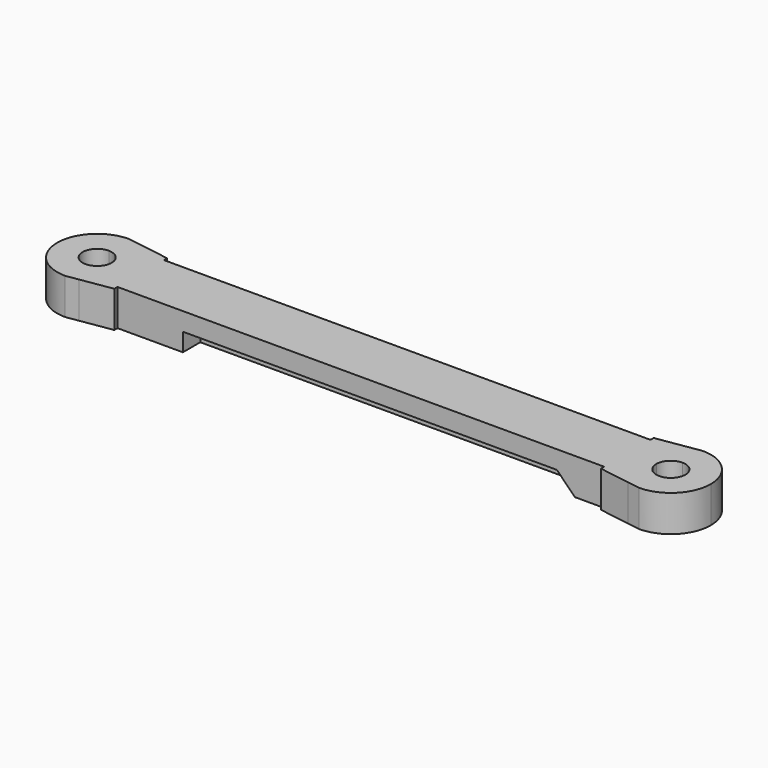
from build123d import *

# Parameters (mm, degrees)
F0_W         = 60
F0_H         = 2
F1_DEPTH     = 5
F2_W         = 9
F2_H         = 3
F3_DEPTH     = 5
F4_W         = 49
F4_H         = 3
F5_DEPTH     = 2.5
F6_T4_DEPTH  = 15.8584149398
F6_T9_DEPTH  = 28.7168298797
F6_T15_DEPTH = 28.7168298797
F6_T21_DEPTH = 15.8584149398


# Not quite as in the source:
# - a fillet or chamfer that OpenCascade refuses, or shapes differently, is made with other operations: its cross-section is extruded or revolved along the edge and cut away or added


with BuildPart() as f1:
    # F0 (on Top) → F1 (new body)
    with BuildSketch(Plane.XY):
        with BuildLine():
            ThreePointArc((21.3155073225, 23.6537444443), (19.7045946191, 27.5428317408), (15.8155073225, 29.1537444443))
            Line((15.8155073225, 29.1537444443), (15.8155073225, 25.6537444443))
            ThreePointArc((15.8155073225, 25.6537444443), (17.2297208849, 25.0679580066), (17.8155073225, 23.6537444443))
            ThreePointArc((17.8155073225, 23.6537444443), (17.2297208849, 22.2395308819), (15.8155073225, 21.6537444443))
            Line((15.8155073225, 21.6537444443), (15.8155073225, 18.1537444443))
            ThreePointArc((15.8155073225, 18.1537444443), (19.7045946191, 19.7646571477), (21.3155073225, 23.6537444443))
        make_face()
        with BuildLine():
            Line((15.8155073225, 29.1537444443), (14.120912728, 28.8861768767))
            ThreePointArc((14.120912728, 28.8861768767), (11.3674588589, 26.8886887815), (10.3155073225, 23.6537444443))
            Line((10.3155073225, 23.6537444443), (13.8155073225, 23.6537444443))
            ThreePointArc((13.8155073225, 23.6537444443), (14.4012937602, 25.0679580066), (15.8155073225, 25.6537444443))
            Line((15.8155073225, 25.6537444443), (15.8155073225, 29.1537444443))
        make_face()
        with BuildLine():
            Line((13.8155073225, 23.6537444443), (10.3155073225, 23.6537444443))
            ThreePointArc((10.3155073225, 23.6537444443), (11.3674588589, 20.418800107), (14.120912728, 18.4213120118))
            Line((14.120912728, 18.4213120118), (15.8155073225, 18.1537444443))
            Line((15.8155073225, 18.1537444443), (15.8155073225, 21.6537444443))
            ThreePointArc((15.8155073225, 21.6537444443), (14.4012937602, 22.2395308819), (13.8155073225, 23.6537444443))
        make_face()
        with BuildLine():
            Line((14.120912728, 28.8861768767), (9.8155073225, 28.2063760232))
            Line((9.8155073225, 28.2063760232), (9.8155073225, 24.6537444443))
            Line((9.8155073225, 24.6537444443), (9.8155073225, 23.6537444443))
            Line((9.8155073225, 23.6537444443), (10.3155073225, 23.6537444443))
            ThreePointArc((10.3155073225, 23.6537444443), (11.3674588589, 26.8886887815), (14.120912728, 28.8861768767))
        make_face()
        with BuildLine():
            Line((10.3155073225, 23.6537444443), (9.8155073225, 23.6537444443))
            Line((9.8155073225, 23.6537444443), (9.8155073225, 22.6537444443))
            Line((9.8155073225, 22.6537444443), (9.8155073225, 19.1011128653))
            Line((9.8155073225, 19.1011128653), (14.120912728, 18.4213120118))
            ThreePointArc((14.120912728, 18.4213120118), (11.3674588589, 20.418800107), (10.3155073225, 23.6537444443))
        make_face()
        with Locations((-23.6844926775, 23.6537444443)):
            Rectangle(F0_W, F0_H)
        Polygon((9.8155073225, 24.6537444443), (6.3155073225, 24.6537444443), (6.3155073225, 22.6537444443), (9.8155073225, 22.6537444443), (9.8155073225, 23.6537444443), align=None)
        with BuildLine():
            ThreePointArc((-57.6844926775, 23.6537444443), (-58.7364442138, 26.8886887815), (-61.4898980829, 28.8861768767))
            Line((-61.4898980829, 28.8861768767), (-63.1844926775, 29.1537444443))
            Line((-63.1844926775, 29.1537444443), (-63.1844926775, 25.6537444443))
            ThreePointArc((-63.1844926775, 25.6537444443), (-61.7702791151, 25.0679580066), (-61.1844926775, 23.6537444443))
            Line((-61.1844926775, 23.6537444443), (-57.6844926775, 23.6537444443))
        make_face()
        with BuildLine():
            ThreePointArc((-61.4898980829, 18.4213120118), (-58.7364442138, 20.418800107), (-57.6844926775, 23.6537444443))
            Line((-57.6844926775, 23.6537444443), (-61.1844926775, 23.6537444443))
            ThreePointArc((-61.1844926775, 23.6537444443), (-61.7702791151, 22.2395308819), (-63.1844926775, 21.6537444443))
            Line((-63.1844926775, 21.6537444443), (-63.1844926775, 18.1537444443))
            Line((-63.1844926775, 18.1537444443), (-61.4898980829, 18.4213120118))
        make_face()
        with BuildLine():
            Line((-63.1844926775, 25.6537444443), (-63.1844926775, 29.1537444443))
            ThreePointArc((-63.1844926775, 29.1537444443), (-68.6844926775, 23.6537444443), (-63.1844926775, 18.1537444443))
            Line((-63.1844926775, 18.1537444443), (-63.1844926775, 21.6537444443))
            ThreePointArc((-63.1844926775, 21.6537444443), (-65.1844926775, 23.6537444443), (-63.1844926775, 25.6537444443))
        make_face()
        with BuildLine():
            Line((-57.1844926775, 24.6537444443), (-57.1844926775, 28.2063760232))
            Line((-57.1844926775, 28.2063760232), (-61.4898980829, 28.8861768767))
            ThreePointArc((-61.4898980829, 28.8861768767), (-58.7364442138, 26.8886887815), (-57.6844926775, 23.6537444443))
            Line((-57.6844926775, 23.6537444443), (-57.1844926775, 23.6537444443))
            Line((-57.1844926775, 23.6537444443), (-57.1844926775, 24.6537444443))
        make_face()
        with BuildLine():
            Line((-57.1844926775, 22.6537444443), (-57.1844926775, 23.6537444443))
            Line((-57.1844926775, 23.6537444443), (-57.6844926775, 23.6537444443))
            ThreePointArc((-57.6844926775, 23.6537444443), (-58.7364442138, 20.418800107), (-61.4898980829, 18.4213120118))
            Line((-61.4898980829, 18.4213120118), (-57.1844926775, 19.1011128653))
            Line((-57.1844926775, 19.1011128653), (-57.1844926775, 22.6537444443))
        make_face()
        Polygon((-53.6844926775, 22.6537444443), (-53.6844926775, 24.6537444443), (-57.1844926775, 24.6537444443), (-57.1844926775, 23.6537444443), (-57.1844926775, 22.6537444443), align=None)
    extrude(amount=F1_DEPTH)

    # F2 (on face) → F3 (join)
    with BuildSketch(Plane(origin=(0, 0, 0), x_dir=(1, 0, 0), z_dir=(0, 0, -1))):
        with Locations((5.3155073225, -21.1537444443)):
            Rectangle(F2_W, F2_H)
        with Locations((5.3155073225, -26.1537444443)):
            Rectangle(F2_W, F2_H)
        with Locations((-52.6844926775, -21.1537444443)):
            Rectangle(F2_W, F2_H)
        with Locations((-52.6844926775, -26.1537444443)):
            Rectangle(F2_W, F2_H)
    extrude(amount=-F3_DEPTH)

    # F4 (on face) → F5 (join)
    with BuildSketch(Plane.XY.offset(5)):
        with Locations((-23.6844926775, 21.1537444443)):
            Rectangle(F4_W, F4_H)
        with Locations((-23.6844926775, 26.1537444443)):
            Rectangle(F4_W, F4_H)
    extrude(amount=-F5_DEPTH)

    # F6: chamfer of 5 on 2 edges, made by hand


with BuildPart() as f6_tool2:
    # F6_s3 → F6_t4 (new body)
    with BuildSketch(Plane.XZ.offset(-6.7953295044)):
        Polygon((0.8155073225, 5), (5.8155073225, 0), (0.8155073225, 0), align=None)
    extrude(amount=-F6_T4_DEPTH)

    split(bisect_by=Plane.XY.offset(2.5), keep=Keep.BOTTOM)


with BuildPart() as f1_1:
    add(f1.part)

    # F6_t1: cut F6_tool2
    add(f6_tool2.part, mode=Mode.SUBTRACT)


with BuildPart() as f6_tool7:
    # F6_s8 → F6_t9 (new body)
    with BuildSketch(Plane.XZ.offset(-6.7953295044)):
        Polygon((0.8155073225, 5), (5.8155073225, 0), (0.8155073225, 0), align=None)
    extrude(amount=-F6_T9_DEPTH)

    split(bisect_by=Plane.XY.offset(2.5), keep=Keep.BOTTOM)

    split(bisect_by=Plane.XZ.offset(-24.6537444443), keep=Keep.BOTTOM)


with BuildPart() as f1_2:
    add(f1_1.part)

    # F6_t6: cut F6_tool7
    add(f6_tool7.part, mode=Mode.SUBTRACT)


with BuildPart() as f6_tool13:
    # F6_s14 → F6_t15 (new body)
    with BuildSketch(Plane.XZ.offset(-11.7953295044)):
        Polygon((0.8155073225, 5), (5.8155073225, 0), (0.8155073225, 0), align=None)
    extrude(amount=-F6_T15_DEPTH)

    split(bisect_by=Plane.XZ.offset(-22.6537444443), keep=Keep.TOP)

    split(bisect_by=Plane.XY.offset(2.5), keep=Keep.BOTTOM)


with BuildPart() as f1_3:
    add(f1_2.part)

    # F6_t12: cut F6_tool13
    add(f6_tool13.part, mode=Mode.SUBTRACT)


with BuildPart() as f6_tool19:
    # F6_s20 → F6_t21 (new body)
    with BuildSketch(Plane.XZ.offset(-24.6537444443)):
        Polygon((0.8155073225, 5), (5.8155073225, 0), (0.8155073225, 0), align=None)
    extrude(amount=-F6_T21_DEPTH)

    split(bisect_by=Plane.XY.offset(2.5), keep=Keep.BOTTOM)


with BuildPart() as f1_4:
    add(f1_3.part)

    # F6_t18: cut F6_tool19
    add(f6_tool19.part, mode=Mode.SUBTRACT)


solid = f1_4.part
